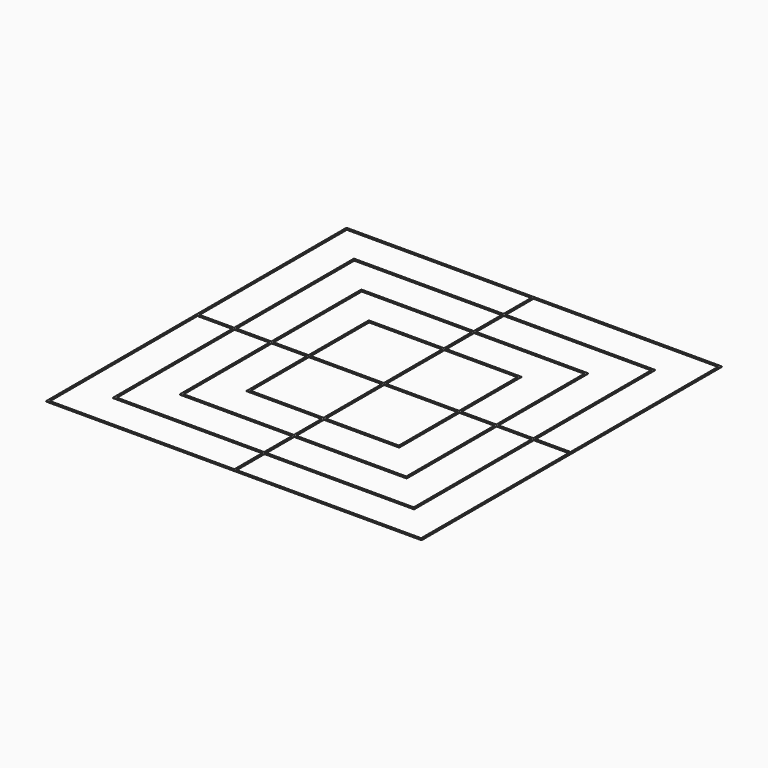
from build123d import *

# Parameters (mm, degrees)
F0_W     = 151.6
F0_H     = 151.6
F0_W_2   = 29.6
F0_H_2   = 0.4
F0_W_3   = 0.4
F0_H_3   = 29.6
F0_W_4   = 14.2
F0_H_4   = 14.2
F0_W_5   = 0.8
F0_H_5   = 0.8
F1_DEPTH = 0.2


with BuildPart() as f1:
    # F0 (on Top) → F1 (new body)
    with BuildSketch(Plane.XY):
        Rectangle(F0_W, F0_H)
        Polygon((75, -0.4), (75, -75), (0.4, -75), (0, -75), (-0.4, -75), (-75, -75), (-75, -0.4), (-75, 0), (-75, 0.4), (-75, 75), (-0.4, 75), (0, 75), (0.4, 75), (75, 75), (75, 0.4), (75, 0), align=None, mode=Mode.SUBTRACT)
        Polygon((-60.8, 60.8), (-60.8, 0.4), (-60, 0.4), (-60, 60), (-0.4, 60), (-0.4, 60.8), align=None)
        Polygon((0.4, -60), (0.4, -60.8), (60.8, -60.8), (60.8, -0.4), (60, -0.4), (60, -60), align=None)
        Polygon((-60.8, -60.8), (-0.4, -60.8), (-0.4, -60), (-60, -60), (-60, -0.4), (-60.8, -0.4), align=None)
        Polygon((60, 0.4), (60.8, 0.4), (60.8, 60.8), (0.4, 60.8), (0.4, 60), (60, 60), align=None)
        Polygon((-45.8, 45.8), (-45.8, 0.4), (-45, 0.4), (-45, 45), (-0.4, 45), (-0.4, 45.8), align=None)
        Polygon((45, 0.4), (45.8, 0.4), (45.8, 45.8), (0.4, 45.8), (0.4, 45), (45, 45), align=None)
        Polygon((-45.8, -45.8), (-0.4, -45.8), (-0.4, -45), (-45, -45), (-45, -0.4), (-45.8, -0.4), align=None)
        Polygon((0.4, -45), (0.4, -45.8), (45.8, -45.8), (45.8, -0.4), (45, -0.4), (45, -45), align=None)
        Polygon((-30.8, 30.8), (-30.8, 0.4), (-30, 0.4), (-30, 30), (-0.4, 30), (-0.4, 30.8), align=None)
        Polygon((-30.8, -30.8), (-0.4, -30.8), (-0.4, -30), (-30, -30), (-30, -0.4), (-30.8, -0.4), align=None)
        Polygon((30, 0.4), (30.8, 0.4), (30.8, 30.8), (0.4, 30.8), (0.4, 30), (30, 30), align=None)
        Polygon((0.4, -30), (0.4, -30.8), (30.8, -30.8), (30.8, -0.4), (30, -0.4), (30, -30), align=None)
        with Locations((15.2, 0.2)):
            Rectangle(F0_W_2, F0_H_2)
        with Locations((-15.2, 0.2)):
            Rectangle(F0_W_2, F0_H_2)
        with Locations((15.2, -0.2)):
            Rectangle(F0_W_2, F0_H_2)
        with Locations((-0.2, 15.2)):
            Rectangle(F0_W_3, F0_H_3)
        with Locations((-15.2, -0.2)):
            Rectangle(F0_W_2, F0_H_2)
        with Locations((-0.2, -15.2)):
            Rectangle(F0_W_3, F0_H_3)
        with Locations((0.2, -15.2)):
            Rectangle(F0_W_3, F0_H_3)
        with Locations((0.2, 15.2)):
            Rectangle(F0_W_3, F0_H_3)
        with Locations((-52.9, -0.2)):
            Rectangle(F0_W_4, F0_H_2)
        with Locations((52.9, -0.2)):
            Rectangle(F0_W_4, F0_H_2)
        with Locations((-37.9, -0.2)):
            Rectangle(F0_W_4, F0_H_2)
        with Locations((67.9, 0.2)):
            Rectangle(F0_W_4, F0_H_2)
        with Locations((-67.9, 0.2)):
            Rectangle(F0_W_4, F0_H_2)
        with Locations((-52.9, 0.2)):
            Rectangle(F0_W_4, F0_H_2)
        with Locations((37.9, 0.2)):
            Rectangle(F0_W_4, F0_H_2)
        with Locations((52.9, 0.2)):
            Rectangle(F0_W_4, F0_H_2)
        with Locations((-37.9, 0.2)):
            Rectangle(F0_W_4, F0_H_2)
        with Locations((0.2, -67.9)):
            Rectangle(F0_W_3, F0_H_4)
        with Locations((-67.9, -0.2)):
            Rectangle(F0_W_4, F0_H_2)
        with Locations((-0.2, 52.9)):
            Rectangle(F0_W_3, F0_H_4)
        with Locations((-0.2, -52.9)):
            Rectangle(F0_W_3, F0_H_4)
        with Locations((0.2, 67.9)):
            Rectangle(F0_W_3, F0_H_4)
        with Locations((67.9, -0.2)):
            Rectangle(F0_W_4, F0_H_2)
        with Locations((0.2, -37.9)):
            Rectangle(F0_W_3, F0_H_4)
        with Locations((0.2, 37.9)):
            Rectangle(F0_W_3, F0_H_4)
        with Locations((37.9, -0.2)):
            Rectangle(F0_W_4, F0_H_2)
        with Locations((0.2, 52.9)):
            Rectangle(F0_W_3, F0_H_4)
        with Locations((-0.2, 37.9)):
            Rectangle(F0_W_3, F0_H_4)
        with Locations((-0.2, -37.9)):
            Rectangle(F0_W_3, F0_H_4)
        with Locations((-0.2, -67.9)):
            Rectangle(F0_W_3, F0_H_4)
        with Locations((-0.2, 67.9)):
            Rectangle(F0_W_3, F0_H_4)
        with Locations((0.2, -52.9)):
            Rectangle(F0_W_3, F0_H_4)
        with Locations((-45.4, 0.2)):
            Rectangle(F0_W_5, F0_H_2)
        with Locations((-60.4, -0.2)):
            Rectangle(F0_W_5, F0_H_2)
        with Locations((30.4, -0.2)):
            Rectangle(F0_W_5, F0_H_2)
        with Locations((-60.4, 0.2)):
            Rectangle(F0_W_5, F0_H_2)
        with Locations((60.4, 0.2)):
            Rectangle(F0_W_5, F0_H_2)
        with Locations((45.4, 0.2)):
            Rectangle(F0_W_5, F0_H_2)
        with Locations((-45.4, -0.2)):
            Rectangle(F0_W_5, F0_H_2)
        with Locations((-30.4, -0.2)):
            Rectangle(F0_W_5, F0_H_2)
        with Locations((-0.2, 45.4)):
            Rectangle(F0_W_3, F0_H_5)
        with Locations((-0.2, -30.4)):
            Rectangle(F0_W_3, F0_H_5)
        with Locations((60.4, -0.2)):
            Rectangle(F0_W_5, F0_H_2)
        with Locations((0.2, 60.4)):
            Rectangle(F0_W_3, F0_H_5)
        with Locations((0.2, -60.4)):
            Rectangle(F0_W_3, F0_H_5)
        with Locations((-30.4, 0.2)):
            Rectangle(F0_W_5, F0_H_2)
        with Locations((30.4, 0.2)):
            Rectangle(F0_W_5, F0_H_2)
        with Locations((-0.2, -60.4)):
            Rectangle(F0_W_3, F0_H_5)
        with Locations((-0.2, 60.4)):
            Rectangle(F0_W_3, F0_H_5)
        with Locations((-0.2, -45.4)):
            Rectangle(F0_W_3, F0_H_5)
        with Locations((0.2, 30.4)):
            Rectangle(F0_W_3, F0_H_5)
        with Locations((0.2, -30.4)):
            Rectangle(F0_W_3, F0_H_5)
        with Locations((45.4, -0.2)):
            Rectangle(F0_W_5, F0_H_2)
        with Locations((0.2, -45.4)):
            Rectangle(F0_W_3, F0_H_5)
        with Locations((0.2, 45.4)):
            Rectangle(F0_W_3, F0_H_5)
        with Locations((-0.2, 30.4)):
            Rectangle(F0_W_3, F0_H_5)
        with Locations((-0.2, 0.2)):
            Rectangle(F0_W_3, F0_H_2)
        with Locations((-0.2, -0.2)):
            Rectangle(F0_W_3, F0_H_2)
        with Locations((0.2, 0.2)):
            Rectangle(F0_W_3, F0_H_2)
        with Locations((0.2, -0.2)):
            Rectangle(F0_W_3, F0_H_2)
    extrude(amount=F1_DEPTH)


solid = f1.part
